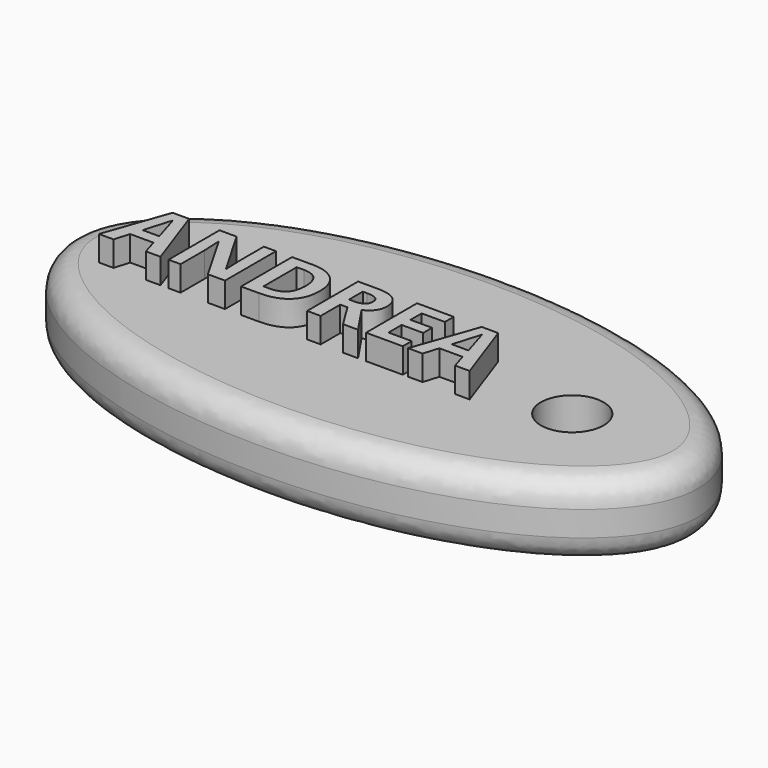
from build123d import *

# Parameters (mm, degrees)
F0_R         = 2.5
F1_DEPTH     = 6
F2_TEXT_SIZE = 7.1119013224
F3_DEPTH     = 2
F4_R         = 2


# Not quite as in the source:
# - Text() gives the source's letters only with a copy of the font that has no kerning and outlines rounded to 1/6400 em; it was checked with that copy


with BuildPart() as f1:
    # F0 (on Top) → F1 (new body)
    with BuildSketch(Plane.XY):
        with BuildLine():
            add(Edge.make_bspline(
                [(28.0115414411, 0), (28.0115414411, 21.6506350946), (-9.4884585589, 10.8253175473), (-46.9884585589, 0), (-9.4884585589, -10.8253175473), (28.0115414411, -21.6506350946), (28.0115414411, 0)],
                knots=[0, 0, 0, 2.0943951024, 2.0943951024, 4.1887902048, 4.1887902048, 6.2831853072, 6.2831853072, 6.2831853072], degree=2, weights=[1, 0.5, 1, 0.5, 1, 0.5, 1]))
        make_face()
        with Locations((18.0115414411, 0)):
            Circle(F0_R, mode=Mode.SUBTRACT)
    extrude(amount=F1_DEPTH)

    # F2 (on face) → F3 (join)
    with BuildSketch(Plane.XY.offset(6)):
        with Locations((-17.7222506945, -2.4776508533)):
            Text('ANDREA', F2_TEXT_SIZE, font='Open Sans', font_style=FontStyle.BOLD, text_align=(TextAlign.LEFT, TextAlign.BOTTOM))
    extrude(amount=F3_DEPTH)

    # F4
    f4_edges = [f1.edges().sort_by_distance(p)[0] for p in [
        (-21.988459, 3e-06, 6),
        (-21.988459, 3e-06, 0),
    ]]
    fillet(f4_edges, radius=F4_R)


solid = f1.part
